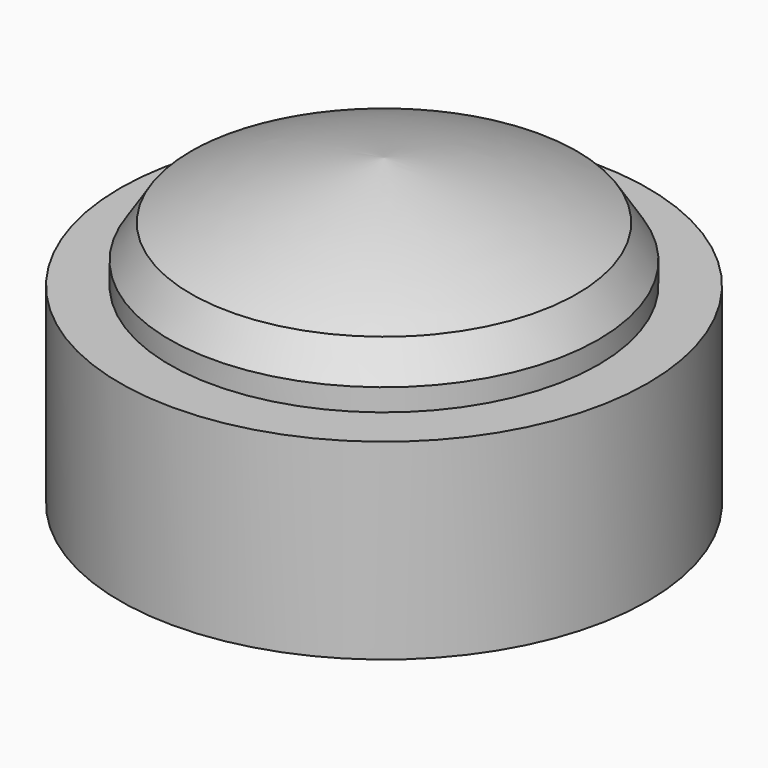
from build123d import *

# Parameters (mm, degrees)
F0_R        = 11.7
F0_R_2      = 10.5
F1_DEPTH    = 8.5
F2_DEPTH    = 7.5
F3_R        = 9.5
F4_DEPTH    = 2
F7_T2_ANGLE = 180
F7_T4_ANGLE = 180


# Not quite as in the source:
# - a fillet or chamfer that OpenCascade refuses, or shapes differently, is made with other operations: its cross-section is extruded or revolved along the edge and cut away or added
# - a feature names something its author has since deleted; it is built from what else it names


with BuildPart() as f1:
    # F0 (on Top) → F1 (new body)
    with BuildSketch(Plane.XY):
        Circle(F0_R)
        Circle(F0_R_2, mode=Mode.SUBTRACT)
        Circle(F0_R_2)
    extrude(amount=F1_DEPTH)

    # F0 (on Top) → F2 (cut)
    with BuildSketch(Plane.XY):
        Circle(F0_R_2)
    extrude(amount=F2_DEPTH, mode=Mode.SUBTRACT)

    # F3 (on face) → F4 (join)
    with BuildSketch(Plane.XY.offset(8.5)):
        Circle(F3_R)
    extrude(amount=F4_DEPTH)

    # F5 (on Front) → F6 (revolve)
    with BuildSketch(Plane.XZ):
        with BuildLine():
            Line((-9.5, 10.5), (0, 10.5))
            Line((0, 10.5), (0, 13.5))
            ThreePointArc((0, 13.5), (-4.8754462608, 12.3972464927), (-9.5, 10.5))
        make_face()
    revolve(axis=Axis((0, 0, 12.3332124203), (0, 0, 1)))

    # F7: chamfer of 1 on 2 edges, made by hand

    # F7_s1 → F7_t2 (revolve, cut)
    with BuildSketch(Plane.XZ):
        with BuildLine():
            Line((-9.5214673898, 9.4467860572), (-8.5368878452, 10.9947550164))
            Line((-8.5368878452, 10.9947550164), (-8.5453666245, 11.0128688316))
            ThreePointArc((-8.5453666245, 11.0128688316), (-9.0246542065, 10.7600809063), (-9.5091067674, 10.5178063693))
            Line((-9.5091067674, 10.5178063693), (-9.52, 10.5))
            ThreePointArc((-9.52, 10.5), (-9.52, 9.9733930286), (-9.5414673898, 9.4467860572))
            Line((-9.5414673898, 9.4467860572), (-9.5214673898, 9.4467860572))
        make_face()
    revolve(axis=Axis((0, 0, 10.5), (0, 0, 1)), revolution_arc=F7_T2_ANGLE, mode=Mode.SUBTRACT)

    # F7_s3 → F7_t4 (revolve, cut)
    with BuildSketch(Plane.XZ):
        with BuildLine():
            Line((9.5214673898, 9.4467860572), (8.5368878452, 10.9947550164))
            Line((8.5368878452, 10.9947550164), (8.5453666245, 11.0128688316))
            ThreePointArc((8.5453666245, 11.0128688316), (9.0246542065, 10.7600809063), (9.5091067674, 10.5178063693))
            Line((9.5091067674, 10.5178063693), (9.52, 10.5))
            ThreePointArc((9.52, 10.5), (9.52, 9.9733930286), (9.5414673898, 9.4467860572))
            Line((9.5414673898, 9.4467860572), (9.5214673898, 9.4467860572))
        make_face()
    revolve(axis=Axis((0, 0, 10.5), (0, 0, 1)), revolution_arc=F7_T4_ANGLE, mode=Mode.SUBTRACT)


solid = f1.part
